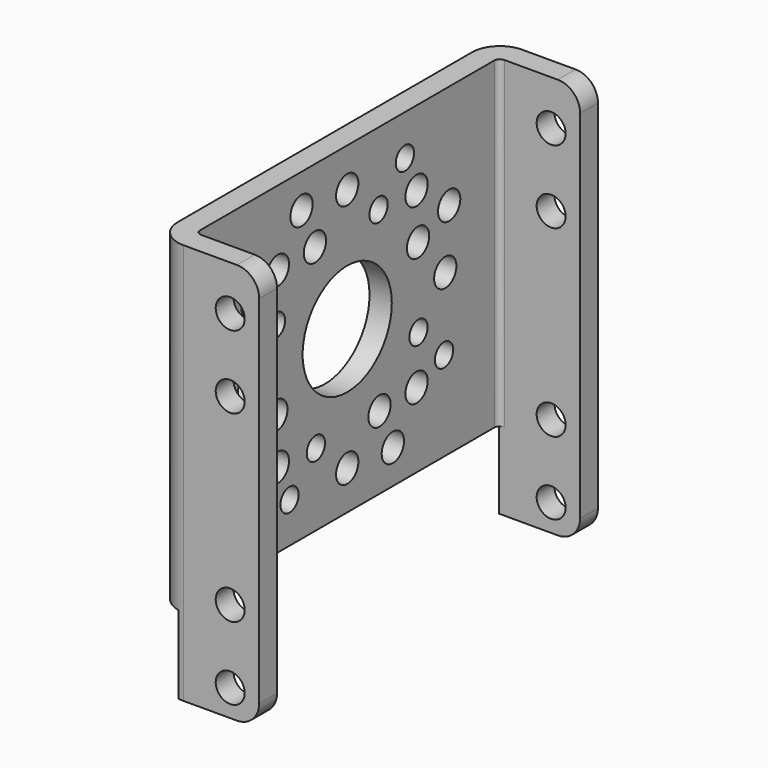
from build123d import *

# Parameters (mm, degrees)
F0_W      = 38
F0_H      = 29
F1_DEPTH  = 2
F2_W      = 2
F2_H      = 36
F3_DEPTH  = 7.3
F4_R      = 2
F5_R      = 0.5
F6_R      = 2.5
F7_R      = 5
F7_R_2    = 1.25
F8_DEPTH  = 25
F9_R      = 1.25
F10_DEPTH = 25
F11_R     = 1.025
F12_DEPTH = 25
F13_R     = 1.25
F14_DEPTH = 25
F15_R     = 1.025
F16_DEPTH = 25
F17_R     = 1.3
F18_DEPTH = 51.6


with BuildPart() as f1:
    # F0 (on Right) → F1 (new body)
    with BuildSketch(Plane.YZ):
        Rectangle(F0_W, F0_H)
    extrude(amount=F1_DEPTH)

    # F2 (on face) → F3 (join)
    with BuildSketch(Plane.YZ.offset(2)):
        with Locations((18, -3.5)):
            Rectangle(F2_W, F2_H)
        with Locations((-18, -3.5)):
            Rectangle(F2_W, F2_H)
    extrude(amount=F3_DEPTH)

    # F4
    f4_edges = [f1.edges().sort_by_distance(p)[0] for p in [
        (9.3, -18, -21.5),
        (9.3, 18, -21.5),
        (9.3, 18, 14.5),
        (9.3, -18, 14.5),
    ]]
    fillet(f4_edges, radius=F4_R)

    # F5
    f5_edges = [f1.edges().sort_by_distance(p)[0] for p in [
        (2, -17, 0),
        (2, 17, 0),
    ]]
    fillet(f5_edges, radius=F5_R)

    # F6
    f6_edges = [f1.edges().sort_by_distance(p)[0] for p in [
        (0, -19, 0),
        (0, 19, 0),
    ]]
    fillet(f6_edges, radius=F6_R)

    # F7 (on face) → F8 (cut)
    with BuildSketch(Plane.YZ.offset(2)):
        Circle(F7_R)
        with Locations((0, -11)):
            Circle(F7_R_2)
        with Locations((7.7781745931, -7.7781745931)):
            Circle(F7_R_2)
        with Locations((11, 0)):
            Circle(F7_R_2)
        with Locations((7.7781745931, 7.7781745931)):
            Circle(F7_R_2)
        with Locations((0, 11)):
            Circle(F7_R_2)
        with Locations((-7.7781745931, 7.7781745931)):
            Circle(F7_R_2)
        with Locations((-11, 0)):
            Circle(F7_R_2)
        with Locations((-7.7781745931, -7.7781745931)):
            Circle(F7_R_2)
    extrude(amount=-F8_DEPTH, mode=Mode.SUBTRACT)

    # F9 (on face) → F10 (cut)
    with BuildSketch(Plane.YZ.offset(2)):
        with Locations((-11.4357154532, -5.1210655213)):
            Circle(F9_R)
        with Locations((5.1210655213, -11.4357154532)):
            Circle(F9_R)
        with Locations((11.4357154532, 5.1210655213)):
            Circle(F9_R)
        with Locations((-5.1210655213, 11.4357154532)):
            Circle(F9_R)
    extrude(amount=-F10_DEPTH, mode=Mode.SUBTRACT)

    # F11 (on face) → F12 (cut)
    with BuildSketch(Plane.YZ.offset(2)):
        with Locations((-7.9929938994, 3.5156610366)):
            Circle(F11_R)
        with Locations((-3.5156610366, -7.9929938994)):
            Circle(F11_R)
        with Locations((7.9929938994, -3.5156610366)):
            Circle(F11_R)
        with Locations((3.5156610366, 7.9929938994)):
            Circle(F11_R)
    extrude(amount=-F12_DEPTH, mode=Mode.SUBTRACT)

    # F13 (on face) → F14 (cut)
    with BuildSketch(Plane.YZ.offset(2)):
        with Locations((-7.9459964827, -3.6206303175)):
            Circle(F13_R)
        with Locations((3.6206303175, -7.9459964827)):
            Circle(F13_R)
        with Locations((7.9459964827, 3.6206303175)):
            Circle(F13_R)
        with Locations((-3.6206303175, 7.9459964827)):
            Circle(F13_R)
    extrude(amount=-F14_DEPTH, mode=Mode.SUBTRACT)

    # F15 (on face) → F16 (cut)
    with BuildSketch(Plane.YZ.offset(2)):
        with Locations((-10.8599086511, 6.4697190889)):
            Circle(F15_R)
        with Locations((-6.4697190889, -10.8599086511)):
            Circle(F15_R)
        with Locations((10.8599086511, -6.4697190889)):
            Circle(F15_R)
        with Locations((6.4697190889, 10.8599086511)):
            Circle(F15_R)
    extrude(amount=-F16_DEPTH, mode=Mode.SUBTRACT)

    # F17 (on face) → F18 (cut)
    with BuildSketch(Plane.XZ.offset(19)):
        with Locations((6.7, 10.469)):
            Circle(F17_R)
        with Locations((6.7, 3.924)):
            Circle(F17_R)
        with Locations((6.7, -12.546)):
            Circle(F17_R)
        with Locations((6.7, -19.091)):
            Circle(F17_R)
    extrude(amount=-F18_DEPTH, mode=Mode.SUBTRACT)


solid = f1.part
